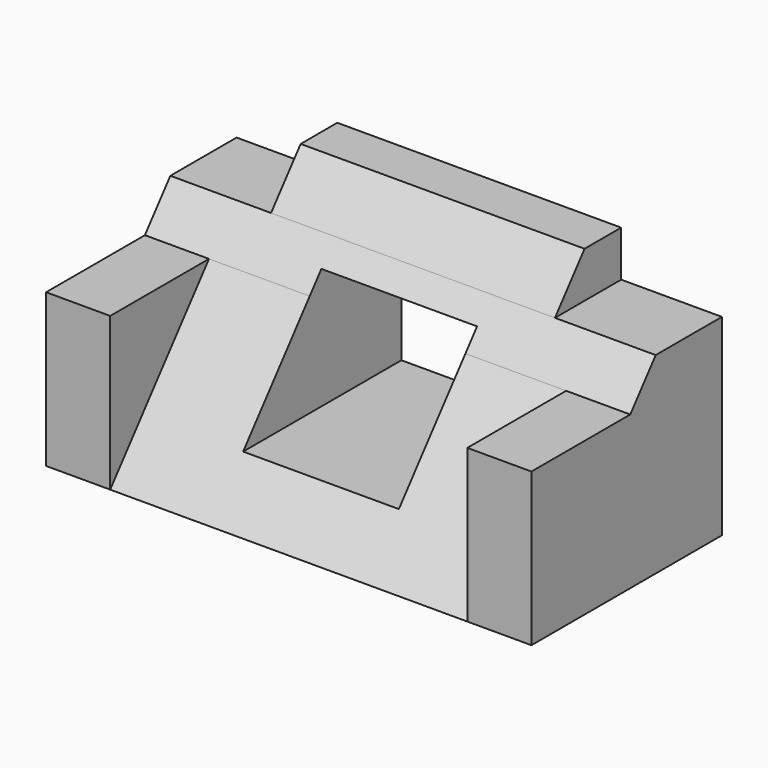
from build123d import *

# Parameters (mm, degrees)
F0_W      = 53
F0_H      = 26
F1_DEPTH  = 26
F3_DEPTH  = 53.001
F4_DEPTH  = 7
F5_DEPTH  = 11
F12_W     = 17
F12_H     = 13.2250000635
F13_DEPTH = 43.9209094299


# Not quite as in the source:
# - a pattern or mirror of a feature is missing from the dataset's text; its kind, count and spacing are read off the source's solid


with BuildPart() as f1:
    # F0 (on Top) → F1 (new body)
    with BuildSketch(Plane.XY):
        Rectangle(F0_W, F0_H)
    extrude(amount=F1_DEPTH)

    # F2 (on face) → F3 (cut, through all)
    with BuildSketch(Plane.YZ.offset(26.5)):
        Polygon((3.9615384615, 21), (8, 26), (-13, 26), (-13, 16.7), (0.4884615385, 16.7), align=None)
        Polygon((0.4884615385, 16.7), (-13, 16.7), (-13, 0), align=None)
    extrude(amount=-F3_DEPTH, mode=Mode.SUBTRACT)

    # F2 (on face) → F4 (join)
    with BuildSketch(Plane.YZ.offset(26.5)):
        Polygon((0.4884615385, 16.7), (-13, 16.7), (-13, 0), align=None)
    f4 = extrude(amount=-F4_DEPTH)

    # F4_copies: F4 across plane
    add(f4.mirror(Plane(origin=(0, 0, 0), x_dir=(0, 0, -1), z_dir=(-1, 0, 0))))

    # F2 (on face) → F5 (cut)
    with BuildSketch(Plane.YZ.offset(26.5)):
        Polygon((13, 21), (13, 26), (8, 26), (3.9615384615, 21), align=None)
    f5 = extrude(amount=-F5_DEPTH, mode=Mode.SUBTRACT)

    # F5_copies: F5 across plane
    add(f5.mirror(Plane(origin=(0, 0, 0), x_dir=(0, 0, -1), z_dir=(-1, 0, 0))), mode=Mode.SUBTRACT)

    # F12 (on 3pt) → F13 (cut, through all)
    with BuildSketch(Plane(origin=(0, -30.9199094299, 0), x_dir=(-1, 0, 0), z_dir=(0, 1, 0))):
        with Locations((0, 12.0580882932)):
            Rectangle(F12_W, F12_H)
    extrude(amount=F13_DEPTH, mode=Mode.SUBTRACT)


solid = f1.part
